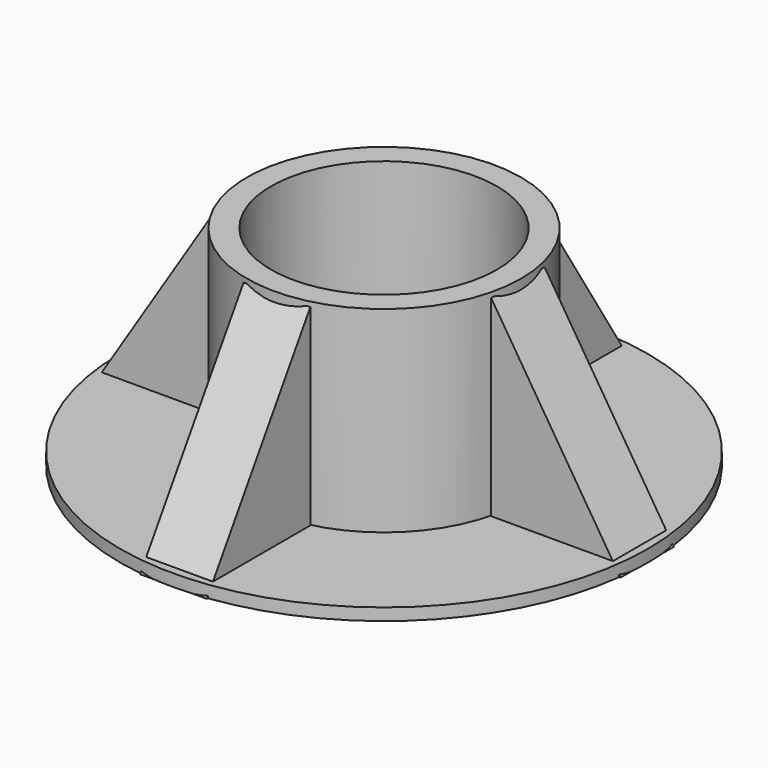
from build123d import *

# Parameters (mm, degrees)
F4_DEPTH        = 7.5
F4_COPIES_COUNT = 4


# Not quite as in the source:
# - a pattern or mirror of a feature is missing from the dataset's text; its kind, count and spacing are read off the source's solid


with BuildPart() as f2:
    # F0 (on Front) → F2 (revolve)
    with BuildSketch(Plane.XZ):
        Polygon((9.3577429652, 0), (59.3534484506, 0), (59.3534484506, 2.7155173011), (30.840517953, 2.7155173011), (30.840517953, 46.9396561384), (25.4094842821, 46.9396561384), (25.7850456983, 0.8370543364), (9.3577429652, 0.8370543364), align=None)
    revolve(axis=Axis((0, 0, 37.2192747891), (0, 0, 1)))

    # F3 (on Front) → F4 (join, symmetric)
    with BuildSketch(Plane.XZ):
        Polygon((59.184409678, 0), (30.097162351, 45.9310486913), (30.097162351, 0), align=None)
    f4 = extrude(amount=F4_DEPTH, both=True)

    # F4_copies: F4 ×4 about axis
    f4_copies_axis = Axis((0, 0, 0), (0, 0, 1))
    for i in range(1, F4_COPIES_COUNT):
        add(f4.rotate(f4_copies_axis, i * 360 / F4_COPIES_COUNT))


solid = f2.part
